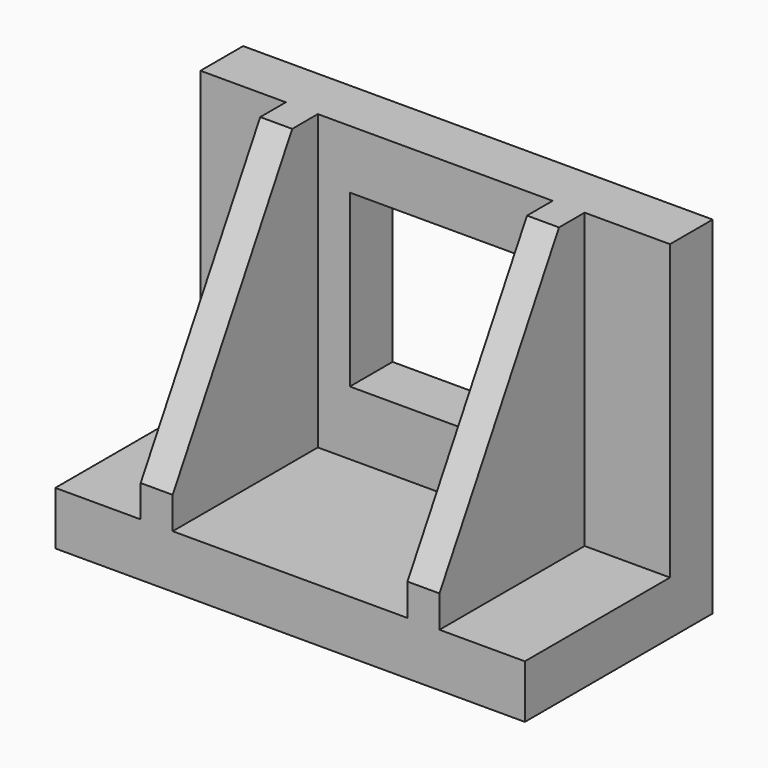
from build123d import *

# Parameters (mm, degrees)
F1_DEPTH = 44
F2_W     = 32
F2_H     = 32
F3_DEPTH = 10.001
F6_DEPTH = 3


# Not quite as in the source:
# - a pattern or mirror of a feature is missing from the dataset's text; its kind, count and spacing are read off the source's solid


with BuildPart() as f1:
    # F0 (on Right) → F1 (new body, symmetric)
    with BuildSketch(Plane.YZ):
        Polygon((0, 10), (0, 0), (44, 0), (44, 65), (34, 65), (34, 10), align=None)
    extrude(amount=F1_DEPTH, both=True)

    # F2 (on face) → F3 (cut, through all)
    with BuildSketch(Plane.XZ.offset(-34)):
        with Locations((0, 38)):
            Rectangle(F2_W, F2_H)
    extrude(amount=-F3_DEPTH, mode=Mode.SUBTRACT)

    # F5 (on offset) → F6 (join, symmetric)
    with BuildSketch(Plane.YZ.offset(25)):
        Polygon((34, 65), (28, 65), (0, 16), (0, 10), (34, 10), align=None)
    f6 = extrude(amount=F6_DEPTH, both=True)

    # F6_copies: F6 across plane
    add(f6.mirror(Plane(origin=(0, 0, 0), x_dir=(0, 0, -1), z_dir=(-1, 0, 0))))


solid = f1.part
